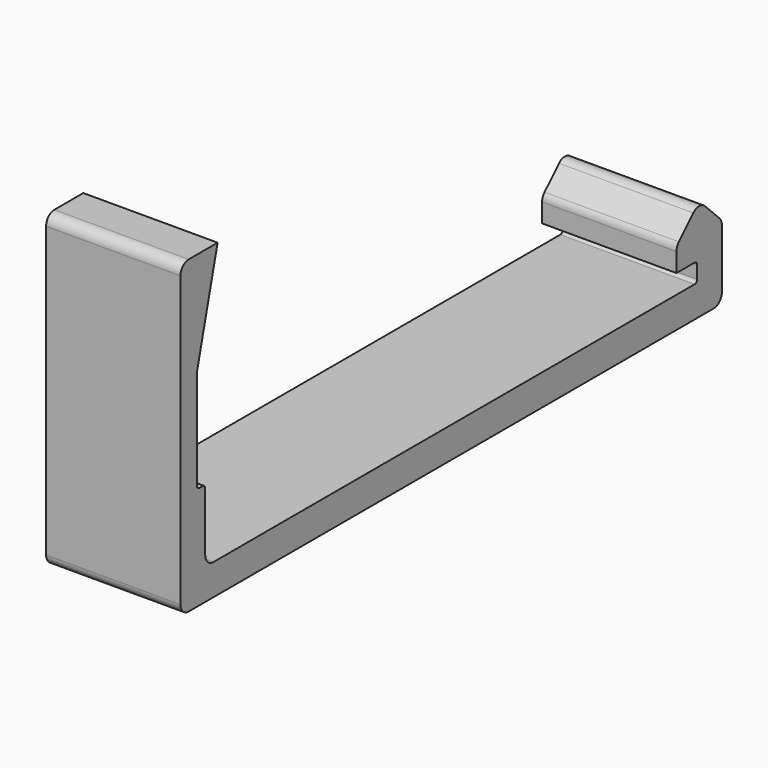
from build123d import *

# Parameters (mm, degrees)
F2_DEPTH = 6.5
F3_R     = 1
F4_R     = 0.3


with BuildPart() as f2:
    # F1 (on Right) → F2 (new body, symmetric)
    with BuildSketch(Plane.YZ):
        Polygon((59.5, 0), (0, 0), (0, 7), (-1, 7), (-1, 17), (1.5, 27), (-3, 27), (-3, -3), (0, -3), (59.5, -3), (62.5, -3), (62.5, 4.1), (59.75, 6.85), (57, 4.1), (57, 1.85), (59.5, 1.85), align=None)
    extrude(amount=F2_DEPTH, both=True)

    # F3
    f3_edges = [f2.edges().sort_by_distance(p)[0] for p in [
        (0, 62.5, -3),
        (0, -3, -3),
        (0, -3, 27),
        (0, 62.5, 4.1),
        (0, 59.75, 6.85),
        (0, 57, 4.1),
        (0, 0, 0),
    ]]
    fillet(f3_edges, radius=F3_R)

    # F4
    f4_edges = [f2.edges().sort_by_distance(p)[0] for p in [
        (0, -1, 17),
        (0, 59.5, 0),
        (0, 59.5, 1.85),
        (0, 0, 7),
        (0, -1, 7),
    ]]
    fillet(f4_edges, radius=F4_R)


solid = f2.part
